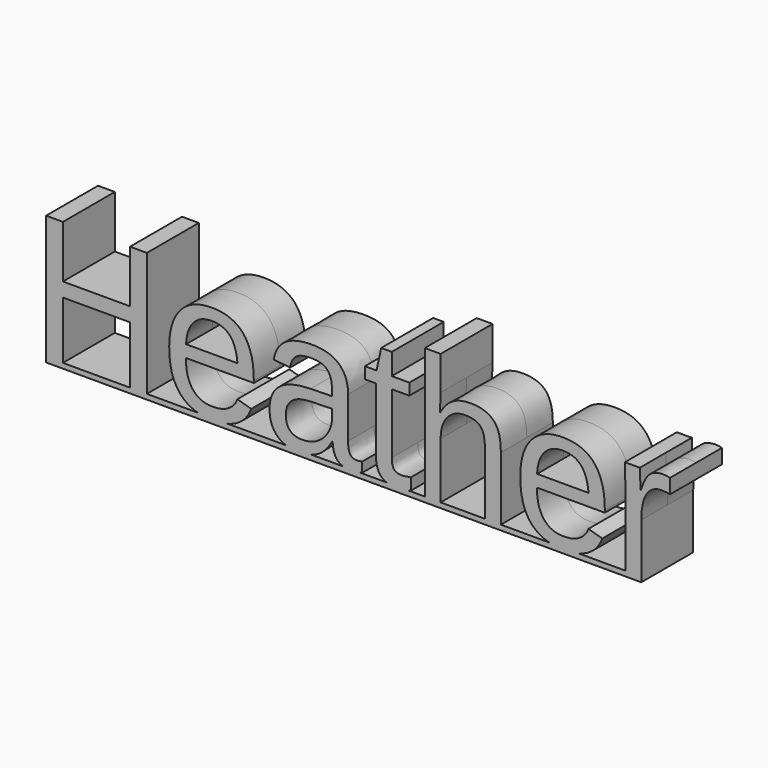
from build123d import *

# Parameters (mm, degrees)
F0_TEXT_SIZE = 35.2777777778
F1_DEPTH     = 6.35
F2_W         = 116.4001302083
F2_H         = 12.7
F3_DEPTH     = 1


# Not quite as in the source:
# - Text() gives the source's letters only with a copy of the font that has no kerning and outlines rounded to 1/6400 em; it was checked with that copy


with BuildPart() as f1:
    # F0 (on Front) → F1 (new body, symmetric)
    with BuildSketch(Plane.XZ):
        with Locations((-63.6791449653, 0)):
            Text('Heather', F0_TEXT_SIZE, font='Arimo', text_align=(TextAlign.LEFT, TextAlign.BOTTOM))
    extrude(amount=F1_DEPTH, both=True)

    # F2 (on Top) → F3 (join)
    with BuildSketch(Plane.XY):
        with Locations((-2.5851996528, 0)):
            Rectangle(F2_W, F2_H)
    extrude(amount=-F3_DEPTH)


solid = f1.part
